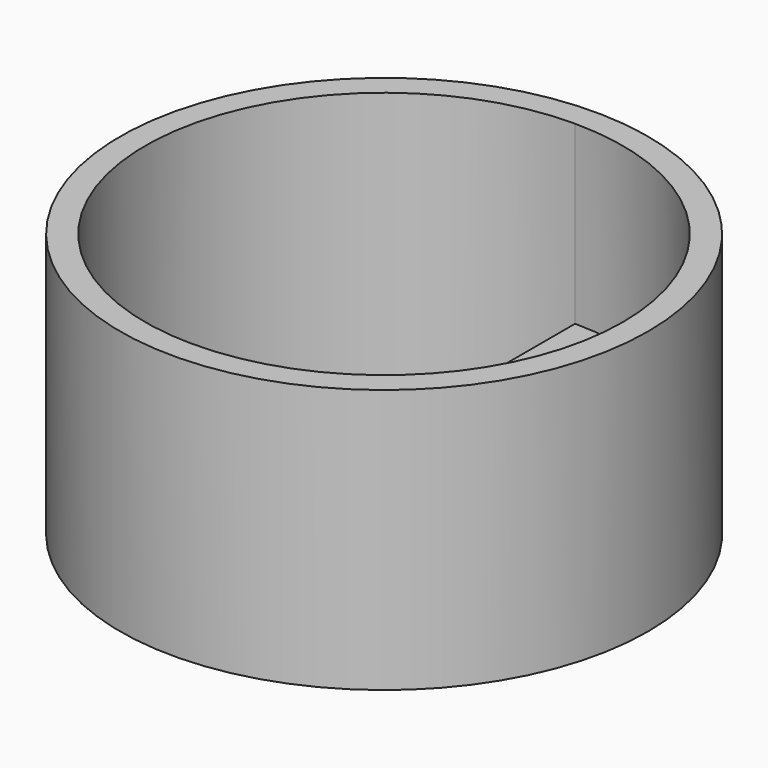
from build123d import *

# Parameters (mm, degrees)
F0_R     = 9.5191370384
F1_DEPTH = 3.175
F2_R     = 9.5191370384
F3_DEPTH = 6.35


with BuildPart() as f1:
    # F0 (on Top) → F1 (new body)
    with BuildSketch(Plane.XY):
        Circle(F0_R)
        with BuildLine():
            ThreePointArc((0, 8.6135921563), (6.0907294241, 6.0907294241), (8.6135921563, 0))
            ThreePointArc((8.6135921563, 0), (6.0907294241, -6.0907294241), (0, -8.6135921563))
            ThreePointArc((0, -8.6135921563), (-8.6135921563, 0), (0, 8.6135921563))
        make_face(mode=Mode.SUBTRACT)
        with BuildLine():
            ThreePointArc((0, -8.6135921563), (6.0907294241, -6.0907294241), (8.6135921563, 0))
            ThreePointArc((8.6135921563, 0), (6.0907294241, 6.0907294241), (0, 8.6135921563))
            Line((0, 8.6135921563), (0, -8.6135921563))
        make_face()
    extrude(amount=F1_DEPTH)

    # F2 (on face) → F3 (join)
    with BuildSketch(Plane.XY.offset(3.175)):
        Circle(F2_R)
        with BuildLine():
            ThreePointArc((0, 8.6092061915), (6.0876280786, 6.0876280786), (8.6092061915, 0))
            ThreePointArc((8.6092061915, 0), (6.0876280786, -6.0876280786), (0, -8.6092061915))
            Line((0, -8.6092061915), (0, -8.6135921563))
            ThreePointArc((0, -8.6135921563), (-8.6135921563, 0), (0, 8.6135921563))
            Line((0, 8.6135921563), (0, 8.6092061915))
        make_face(mode=Mode.SUBTRACT)
    extrude(amount=F3_DEPTH)


solid = f1.part
